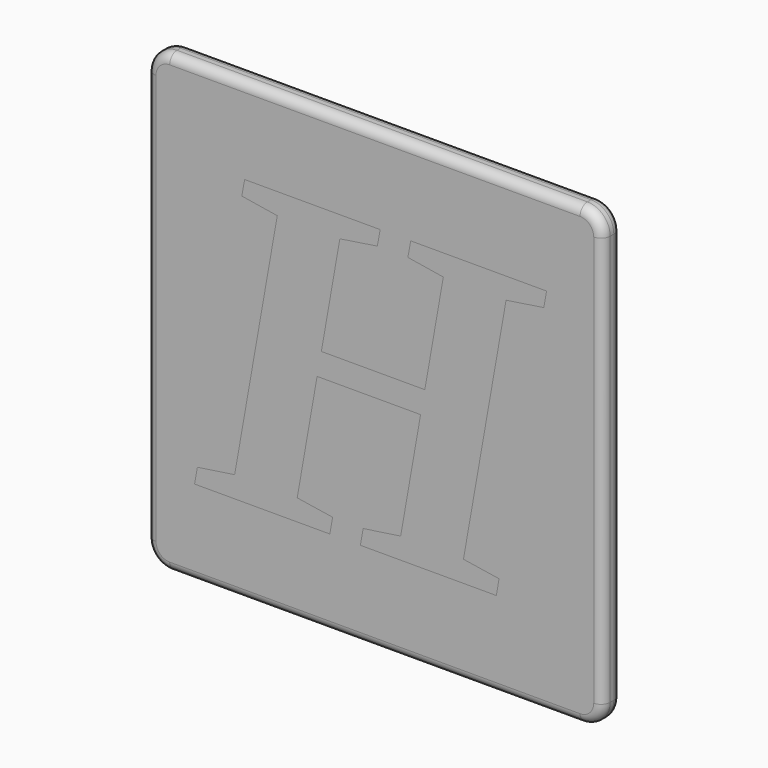
from build123d import *

# Parameters (mm, degrees)
F0_W         = 100
F0_H         = 100
F1_DEPTH     = 5
F2_R         = 5
F3_R         = 2
F4_TEXT_SIZE = 95.2380942181
F5_DEPTH     = 2
F6_DEPTH     = 2


# Not quite as in the source:
# - Text() gives the source's letters only with a copy of the font that has no kerning and outlines rounded to 1/6400 em; it was checked with that copy


with BuildPart() as f1:
    # F0 (on Front) → F1 (new body)
    with BuildSketch(Plane.XZ):
        Rectangle(F0_W, F0_H)
    extrude(amount=F1_DEPTH)

    # F2
    f2_edges = [f1.edges().sort_by_distance(p)[0] for p in [
        (50, -2.5, 50),
        (-50, -2.5, 50),
        (-50, -2.5, -50),
        (50, -2.5, -50),
    ]]
    fillet(f2_edges, radius=F2_R)

    # F3
    f3_edges = [f1.edges().sort_by_distance(p)[0] for p in [
        (50, -5, 0),
        (48.535534, -5, -48.535534),
        (48.535534, -5, 48.535534),
        (0, -5, -50),
        (0, -5, 50),
        (-48.535534, -5, -48.535534),
        (-48.535534, -5, 48.535534),
        (-50, -5, 0),
        (50, 0, 0),
        (48.535534, 0, -48.535534),
        (48.535534, 0, 48.535534),
        (0, 0, -50),
        (0, 0, 50),
        (-48.535534, 0, -48.535534),
        (-48.535534, 0, 48.535534),
        (-50, 0, 0),
    ]]
    fillet(f3_edges, radius=F3_R)

    # F4 (on face) → F5 (cut)
    with BuildSketch(Plane.XZ.offset(5)):
        with Locations((-38.8478841751, -31.1590510374)):
            Text('H', F4_TEXT_SIZE, font='Tinos', font_style=FontStyle.BOLDITALIC, text_align=(TextAlign.LEFT, TextAlign.BOTTOM))
    extrude(amount=-F5_DEPTH, mode=Mode.SUBTRACT)


with BuildPart() as f6:
    # F6 (new): a face of the model
    f6_faces = [f1.part.faces().sort_by_distance(p)[0] for p in [
        (-0.9618810819, -3, 0.0672110721),
    ]]
    extrude(f6_faces, amount=F6_DEPTH)


solid = Compound([f1.part, f6.part])
